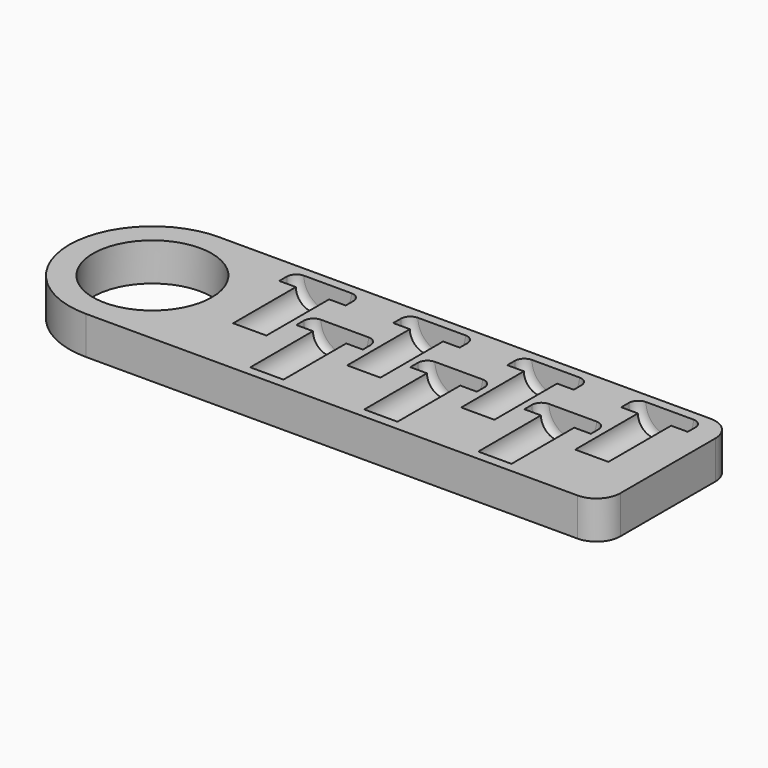
from build123d import *

# Parameters (mm, degrees)
F0_R          = 12.5
F1_DEPTH      = 8
F10_TEXT_SIZE = 5.5555555556
F11_DEPTH     = 1


# Not quite as in the source:
# - Text() gives the source's letters only with a copy of the font that has no kerning and outlines rounded to 1/6400 em; it was checked with that copy


with BuildPart() as f1:
    # F0 (on Top) → F1 (new body)
    with BuildSketch(Plane.XY):
        with BuildLine():
            ThreePointArc((0, 17.5), (5.1256313292, 5.1256313292), (17.5, 0))
            Line((17.5, 0), (121, 0))
            ThreePointArc((121, 0), (124.5355339059, 1.4644660941), (126, 5))
            Line((126, 5), (126, 30))
            ThreePointArc((126, 30), (124.5355339059, 33.5355339059), (121, 35))
            Line((121, 35), (17.5, 35))
            ThreePointArc((17.5, 35), (5.1256313292, 29.8743686708), (0, 17.5))
        make_face()
        with Locations((17.5, 17.5)):
            Circle(F0_R, mode=Mode.SUBTRACT)
    extrude(amount=F1_DEPTH)

    # F2 (on face) → F3 (revolve, cut)
    with BuildSketch(Plane.XY.offset(8)):
        with BuildLine():
            Line((47, 33), (42, 33))
            Line((42, 33), (42, 29))
            Line((42, 29), (42, 12.5))
            Line((42, 12.5), (45.5, 12.5))
            Line((45.5, 12.5), (45.5, 29))
            Line((45.5, 29), (49, 29))
            Line((49, 29), (49, 31))
            ThreePointArc((49, 31), (48.4142135624, 32.4142135624), (47, 33))
        make_face()
    revolve(axis=Axis((42, 20.75, 8), (0, -1, 0)), mode=Mode.SUBTRACT)

    # F2 (on face) → F4 (revolve, cut)
    with BuildSketch(Plane.XY.offset(8)):
        with BuildLine():
            Line((54, 18.5), (54, 2))
            Line((54, 2), (57.5, 2))
            Line((57.5, 2), (57.5, 18.5))
            Line((57.5, 18.5), (61, 18.5))
            Line((61, 18.5), (61, 20.5))
            ThreePointArc((61, 20.5), (60.4142135624, 21.9142135624), (59, 22.5))
            Line((59, 22.5), (54, 22.5))
            Line((54, 22.5), (54, 18.5))
        make_face()
    revolve(axis=Axis((54, 10.25, 8), (0, 1, 0)), mode=Mode.SUBTRACT)

    # F2 (on face) → F5 (revolve, cut)
    with BuildSketch(Plane.XY.offset(8)):
        with BuildLine():
            Line((71, 33), (66, 33))
            Line((66, 33), (66, 29))
            Line((66, 29), (66, 12.5))
            Line((66, 12.5), (69.5, 12.5))
            Line((69.5, 12.5), (69.5, 29))
            Line((69.5, 29), (73, 29))
            Line((73, 29), (73, 31))
            ThreePointArc((73, 31), (72.4142135624, 32.4142135624), (71, 33))
        make_face()
    revolve(axis=Axis((66, 20.75, 8), (0, -1, 0)), mode=Mode.SUBTRACT)

    # F2 (on face) → F6 (revolve, cut)
    with BuildSketch(Plane.XY.offset(8)):
        with BuildLine():
            Line((78, 18.5), (78, 2))
            Line((78, 2), (81.5, 2))
            Line((81.5, 2), (81.5, 18.5))
            Line((81.5, 18.5), (85, 18.5))
            Line((85, 18.5), (85, 20.5))
            ThreePointArc((85, 20.5), (84.4142135624, 21.9142135624), (83, 22.5))
            Line((83, 22.5), (78, 22.5))
            Line((78, 22.5), (78, 18.5))
        make_face()
    revolve(axis=Axis((78, 10.25, 8), (0, 1, 0)), mode=Mode.SUBTRACT)

    # F2 (on face) → F7 (revolve, cut)
    with BuildSketch(Plane.XY.offset(8)):
        with BuildLine():
            Line((102, 18.5), (102, 2))
            Line((102, 2), (105.5, 2))
            Line((105.5, 2), (105.5, 18.5))
            Line((105.5, 18.5), (109, 18.5))
            Line((109, 18.5), (109, 20.5))
            ThreePointArc((109, 20.5), (108.4142135624, 21.9142135624), (107, 22.5))
            Line((107, 22.5), (102, 22.5))
            Line((102, 22.5), (102, 18.5))
        make_face()
    revolve(axis=Axis((102, 10.25, 8), (0, 1, 0)), mode=Mode.SUBTRACT)

    # F2 (on face) → F8 (revolve, cut)
    with BuildSketch(Plane.XY.offset(8)):
        with BuildLine():
            Line((95, 33), (90, 33))
            Line((90, 33), (90, 29))
            Line((90, 29), (90, 12.5))
            Line((90, 12.5), (93.5, 12.5))
            Line((93.5, 12.5), (93.5, 29))
            Line((93.5, 29), (97, 29))
            Line((97, 29), (97, 31))
            ThreePointArc((97, 31), (96.4142135624, 32.4142135624), (95, 33))
        make_face()
    revolve(axis=Axis((90, 20.75, 8), (0, -1, 0)), mode=Mode.SUBTRACT)

    # F2 (on face) → F9 (revolve, cut)
    with BuildSketch(Plane.XY.offset(8)):
        with BuildLine():
            Line((119, 33), (114, 33))
            Line((114, 33), (114, 29))
            Line((114, 29), (114, 12.5))
            Line((114, 12.5), (117.5, 12.5))
            Line((117.5, 12.5), (117.5, 29))
            Line((117.5, 29), (121, 29))
            Line((121, 29), (121, 31))
            ThreePointArc((121, 31), (120.4142135624, 32.4142135624), (119, 33))
        make_face()
    revolve(axis=Axis((114, 20.75, 8), (0, -1, 0)), mode=Mode.SUBTRACT)

    # F10 (on face) → F11 (cut)
    with BuildSketch(Plane(origin=(0, 0, 0), x_dir=(1, 0, 0), z_dir=(0, 0, -1))):
        with Locations((30, -9)):
            Text('923, 924', F10_TEXT_SIZE, font='Open Sans', text_align=(TextAlign.LEFT, TextAlign.BOTTOM))
    extrude(amount=-F11_DEPTH, mode=Mode.SUBTRACT)


solid = f1.part
